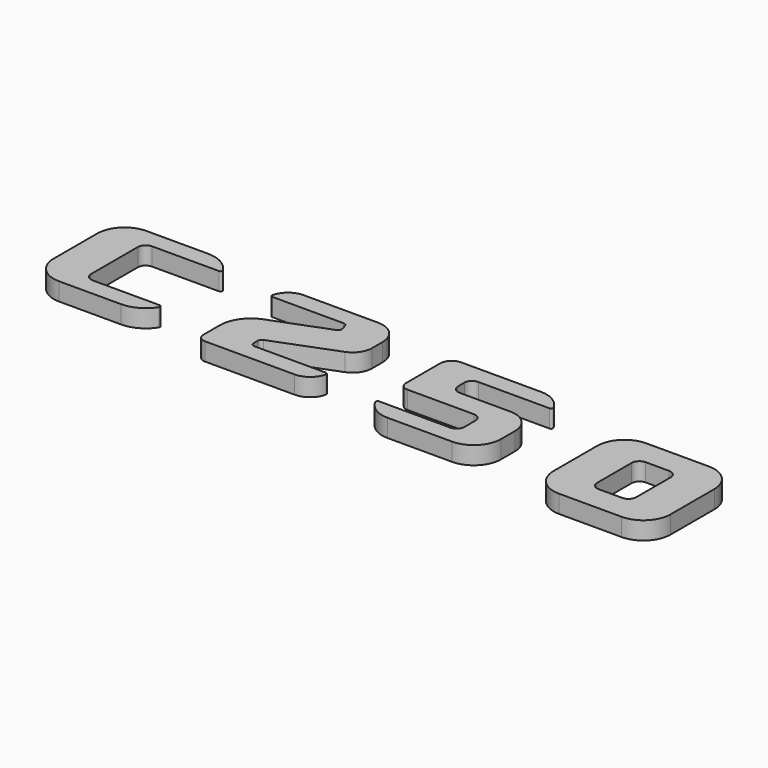
from build123d import *

# Parameters (mm, degrees)
F1_DEPTH     = 4.57
F2_R         = 2
F3_R         = 7
F4_T1_DEPTH  = 40.5387364248
F5_R         = 0.5
F7_DEPTH     = 4.57
F8_T1_DEPTH  = 29.4446859277
F9_R         = 5
F10_R        = 1
F11_R        = 0.5
F12_R        = 2
F13_R        = 8
F14_R        = 6
F16_DEPTH    = 4.57
F17_T1_DEPTH = 37.2617420766
F18_R        = 0.5
F19_R        = 2
F20_R        = 3
F21_R        = 2
F22_R        = 6
F23_R        = 7
F24_W        = 30
F24_H        = 27.94
F24_W_2      = 10
F24_H_2      = 15
F25_DEPTH    = 4.57
F26_R        = 7
F27_R        = 2


# Not quite as in the source:
# - a fillet or chamfer that OpenCascade refuses, or shapes differently, is made with other operations: its cross-section is extruded or revolved along the edge and cut away or added


with BuildPart() as f1:
    # F0 (on Top) → F1 (new body)
    with BuildSketch(Plane.XY):
        Polygon((-24.0826935321, 9.451819914), (-24.0826935321, 13.951819914), (-54.0826935321, 13.951819914), (-54.0826935321, -13.988180086), (-24.0826935321, -13.988180086), (-24.0826935321, -9.488180086), (-44.0826935321, -9.488180086), (-44.0826935321, 9.451819914), align=None)
    extrude(amount=F1_DEPTH)

    # F2
    f2_edges = [f1.edges().sort_by_distance(p)[0] for p in [
        (-44.082694, 9.45182, 2.285),
        (-44.082694, -9.48818, 2.285),
    ]]
    fillet(f2_edges, radius=F2_R)

    # F3
    f3_edges = [f1.edges().sort_by_distance(p)[0] for p in [
        (-54.082694, 13.95182, 2.285),
        (-54.082694, -13.98818, 2.285),
    ]]
    fillet(f3_edges, radius=F3_R)

    # F4: fillet of radius 8 on 2 edges, made by hand

    # F4_s2 → F4_t1 (cut)
    with BuildSketch(Plane.XY.offset(-17.9843682124)):
        with BuildLine():
            ThreePointArc((-31.2764408171, -13.988180086), (-27.03380013, -12.7705100691), (-24.0826935321, -9.488180086))
            Line((-24.0826935321, -9.488180086), (-24.0826935321, -13.988180086))
            Line((-24.0826935321, -13.988180086), (-31.2764408171, -13.988180086))
        make_face()
        with BuildLine():
            ThreePointArc((-31.2764408171, 13.951819914), (-27.03380013, 12.7341498971), (-24.0826935321, 9.451819914))
            Line((-24.0826935321, 9.451819914), (-24.0826935321, 13.951819914))
            Line((-24.0826935321, 13.951819914), (-31.2764408171, 13.951819914))
        make_face()
    extrude(amount=F4_T1_DEPTH, mode=Mode.SUBTRACT)

    # F5
    f5_edges = [f1.edges().sort_by_distance(p)[0] for p in [
        (-24.082694, -9.48818, 2.285),
        (-24.082694, 9.45182, 2.285),
    ]]
    fillet(f5_edges, radius=F5_R)


with BuildPart() as f7:
    # F6 (on Top) → F7 (new body)
    with BuildSketch(Plane.XY):
        Polygon((19.8506022431, 11.8833926581), (-10.1493977569, 11.8833926581), (-10.1493977569, 7.3833926581), (9.3855382875, 7.3833926581), (10.2475822992, 4.5099139089), (-10.1172720553, -3.3282011872), (-10.1172720553, -16.0566073419), (19.8506022431, -16.0566073419), (19.8506022431, -11.5566073419), (0, -11.5566073419), (0, -8.5566073419), (19.8506022431, -0.9029187956), align=None)
    extrude(amount=F7_DEPTH)

    # F8: fillet of radius 5 on 2 edges, made by hand

    # F8_s2 → F8_t1 (cut)
    with BuildSketch(Plane.XY.offset(-12.4373429638)):
        with BuildLine():
            ThreePointArc((14.8756650576, -16.0566073419), (18.2297670238, -14.7647065855), (19.8506022431, -11.5566073419))
            Line((19.8506022431, -11.5566073419), (19.8506022431, -16.0566073419))
            Line((19.8506022431, -16.0566073419), (14.8756650576, -16.0566073419))
        make_face()
        with BuildLine():
            ThreePointArc((-5.1744605714, 11.8833926581), (-8.5285625376, 10.5914919016), (-10.1493977569, 7.3833926581))
            Line((-10.1493977569, 7.3833926581), (-10.1493977569, 11.8833926581))
            Line((-10.1493977569, 11.8833926581), (-5.1744605714, 11.8833926581))
        make_face()
    extrude(amount=F8_T1_DEPTH, mode=Mode.SUBTRACT)

    # F9
    f9_edges = [f7.edges().sort_by_distance(p)[0] for p in [
        (19.850602, -0.902919, 2.285),
    ]]
    fillet(f9_edges, radius=F9_R)

    # F10
    f10_edges = [f7.edges().sort_by_distance(p)[0] for p in [
        (9.385538, 7.383393, 2.285),
        (10.247582, 4.509914, 2.285),
        (0, -8.556607, 2.285),
        (0, -11.556607, 2.285),
    ]]
    fillet(f10_edges, radius=F10_R)

    # F11
    f11_edges = [f7.edges().sort_by_distance(p)[0] for p in [
        (-10.149398, 7.383393, 2.285),
        (19.850602, -11.556607, 2.285),
    ]]
    fillet(f11_edges, radius=F11_R)

    # F12
    f12_edges = [f7.edges().sort_by_distance(p)[0] for p in [
        (-10.117272, -16.056607, 2.285),
    ]]
    fillet(f12_edges, radius=F12_R)

    # F13
    f13_edges = [f7.edges().sort_by_distance(p)[0] for p in [
        (-10.117272, -3.328201, 2.285),
    ]]
    fillet(f13_edges, radius=F13_R)

    # F14
    f14_edges = [f7.edges().sort_by_distance(p)[0] for p in [
        (19.850602, 11.883393, 2.285),
    ]]
    fillet(f14_edges, radius=F14_R)


with BuildPart() as f16:
    # F15 (on Top) → F16 (new body)
    with BuildSketch(Plane.XY):
        Polygon((64.6036404371, 4.3333959766), (64.6036404371, 8.8333959766), (34.6036404371, 8.8333959766), (34.6036404371, -7.1066040234), (55.6036404371, -7.1066040234), (55.6036404371, -14.6066040234), (34.6036404371, -14.6066040234), (34.6036404371, -19.1066040234), (64.6036404371, -19.1066040234), (64.6036404371, -1.6666040234), (43.6036404371, -1.6666040234), (43.6036404371, 4.3333959766), align=None)
    extrude(amount=F16_DEPTH)

    # F17: fillet of radius 7 on 2 edges, made by hand

    # F17_s2 → F17_t1 (cut)
    with BuildSketch(Plane.XY.offset(-16.3458710383)):
        with BuildLine():
            ThreePointArc((34.6036404371, -14.6066040234), (37.1733618858, -17.8728853208), (41.1419888524, -19.1066040234))
            Line((41.1419888524, -19.1066040234), (34.6036404371, -19.1066040234))
            Line((34.6036404371, -19.1066040234), (34.6036404371, -14.6066040234))
        make_face()
        with BuildLine():
            ThreePointArc((64.6036404371, 4.3333959766), (62.0339189884, 7.5996772739), (58.0652920218, 8.8333959766))
            Line((58.0652920218, 8.8333959766), (64.6036404371, 8.8333959766))
            Line((64.6036404371, 8.8333959766), (64.6036404371, 4.3333959766))
        make_face()
    extrude(amount=F17_T1_DEPTH, mode=Mode.SUBTRACT)

    # F18
    f18_edges = [f16.edges().sort_by_distance(p)[0] for p in [
        (34.60364, -14.606604, 2.285),
        (64.60364, 4.333396, 2.285),
    ]]
    fillet(f18_edges, radius=F18_R)

    # F19
    f19_edges = [f16.edges().sort_by_distance(p)[0] for p in [
        (55.60364, -7.106604, 2.285),
        (55.60364, -14.606604, 2.285),
        (43.60364, -1.666604, 2.285),
        (43.60364, 4.333396, 2.285),
    ]]
    fillet(f19_edges, radius=F19_R)

    # F20
    f20_edges = [f16.edges().sort_by_distance(p)[0] for p in [
        (34.60364, 8.833396, 2.285),
    ]]
    fillet(f20_edges, radius=F20_R)

    # F21
    f21_edges = [f16.edges().sort_by_distance(p)[0] for p in [
        (34.60364, -7.106604, 2.285),
    ]]
    fillet(f21_edges, radius=F21_R)

    # F22
    f22_edges = [f16.edges().sort_by_distance(p)[0] for p in [
        (64.60364, -1.666604, 2.285),
    ]]
    fillet(f22_edges, radius=F22_R)

    # F23
    f23_edges = [f16.edges().sort_by_distance(p)[0] for p in [
        (64.60364, -19.106604, 2.285),
    ]]
    fillet(f23_edges, radius=F23_R)


with BuildPart() as f25:
    # F24 (on Top) → F25 (new body)
    with BuildSketch(Plane.XY):
        with Locations((96.4378112555, -9.3873783189)):
            Rectangle(F24_W, F24_H)
        with Locations((96.4378112555, -9.3873783189)):
            Rectangle(F24_W_2, F24_H_2, mode=Mode.SUBTRACT)
    extrude(amount=F25_DEPTH)

    # F26
    f26_edges = [f25.edges().sort_by_distance(p)[0] for p in [
        (81.437811, -23.357378, 2.285),
        (111.437811, -23.357378, 2.285),
        (111.437811, 4.582622, 2.285),
        (81.437811, 4.582622, 2.285),
    ]]
    fillet(f26_edges, radius=F26_R)

    # F27
    f27_edges = [f25.edges().sort_by_distance(p)[0] for p in [
        (91.437811, -1.887378, 2.285),
        (101.437811, -1.887378, 2.285),
        (101.437811, -16.887378, 2.285),
        (91.437811, -16.887378, 2.285),
    ]]
    fillet(f27_edges, radius=F27_R)


solid = Compound([f1.part, f7.part, f16.part, f25.part])
